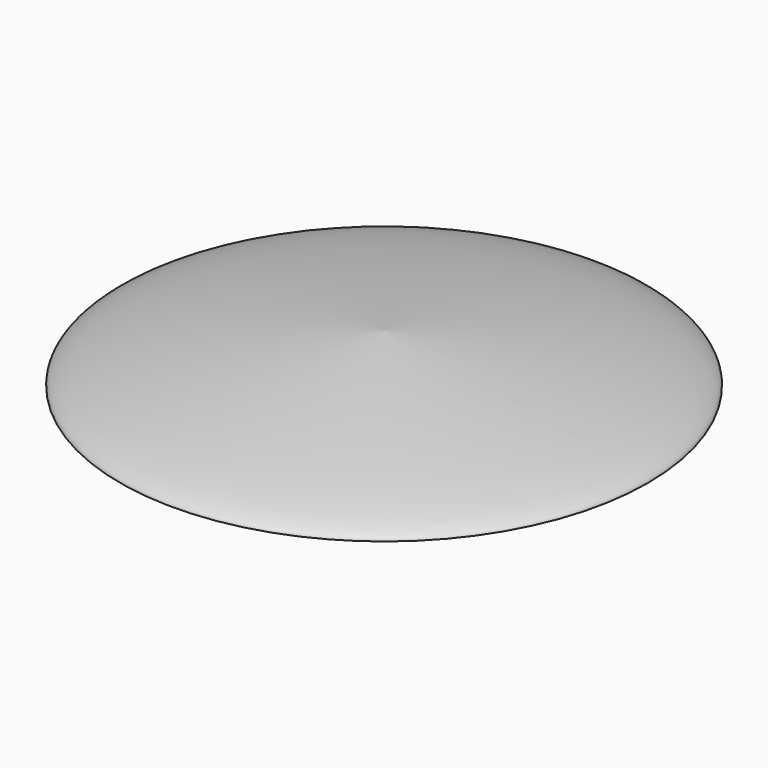
from build123d import *

# Parameters (mm, degrees)
F2_T = 5


# Not quite as in the source:
# - a shell that OpenCascade refuses in one call is made with other operations: the cavity is built on its own and cut out


with BuildPart() as f1:
    # F0 (on Front) → F1 (revolve)
    with BuildSketch(Plane.XZ):
        with BuildLine():
            Line((0, 60), (0, 0))
            Line((0, 0), (330.2, 0))
            Line((330.2, 0), (330.2, 0.491212571))
            add(Edge.make_bspline(
                [(330.2, 0.491212571), (330.1980437316, 0.5130971248), (330.1957416501, 0.5350125601)],
                knots=[0.0163739353, 0.0163739353, 0.0163739353, 0.0178212018, 0.0178212018, 0.0178212018], degree=2, weights=[1, 0.9999997382, 1]))
            add(Edge.make_bspline(
                [(330.1957416501, 0.5350125601), (327.0449626403, 30.5299073872), (0, 60)],
                knots=[0.0178212018, 0.0178212018, 0.0178212018, 1.5789832944, 1.5789832944, 1.5789832944], degree=2, weights=[1, 0.7105047801, 1]))
        make_face()
    revolve(axis=Axis((0, 0, 12.8723818064), (0, 0, -1)))

    # F2: shell of thickness 5, made by hand


with BuildPart() as f2_core1:
    # F2_t2: copy of F1
    add(f1.part)

    # the walls: a layer under each face that stays
    f2_faces = [f2_core1.faces().sort_by_distance(p)[0] for p in [
        (-330.2, 0, 0.2456062855),
        (-330.1979572783, 0, 0.5131048452),
        (-232.3670092676, 0, 30.3765017316),
    ]]
    thicken(f2_faces, amount=-F2_T, mode=Mode.SUBTRACT)


with BuildPart() as f1_1:
    add(f1.part)

    # what is left inside the walls is the cavity
    f2_cavity = [f2_core1.part.solids().sort_by_distance(p)[0] for p in [
        (-272.941603, 0, 17.11474),
    ]]
    add(f2_cavity, mode=Mode.SUBTRACT)


solid = f1_1.part
